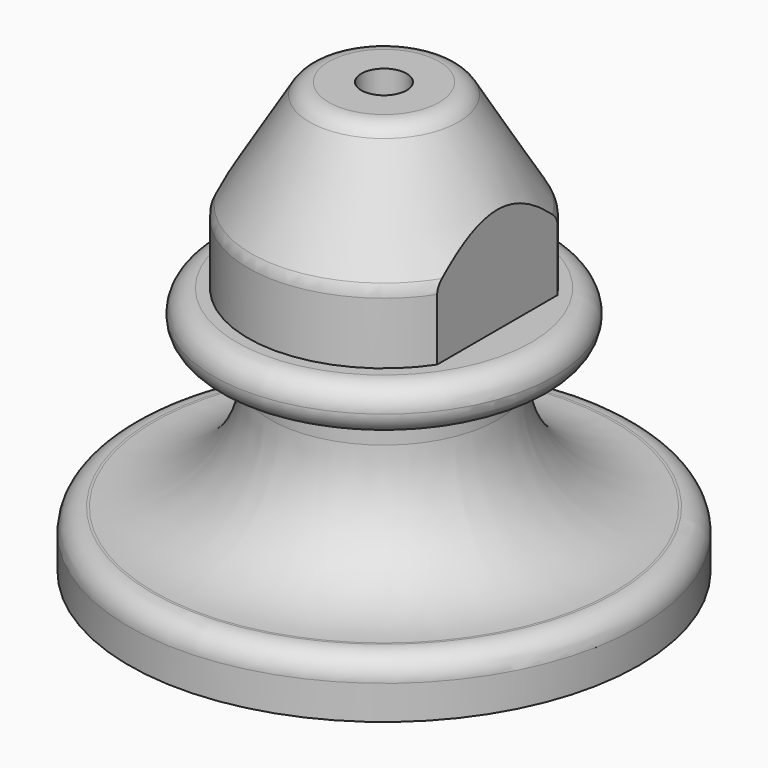
from build123d import *

# Parameters (mm, degrees)
F2_R     = 2
F3_R     = 2
F5_DEPTH = 16
F6_R     = 1.99999


# Not quite as in the source:
# - a fillet or chamfer is up to 0.001 mm smaller than in the source, because OpenCascade refuses the exact size


with BuildPart() as f1:
    # F0 (on Front) → F1 (revolve)
    with BuildSketch(Plane.XZ):
        with BuildLine():
            Line((19.5, 2.4493911769), (19.5, 0))
            Line((19.5, 0), (22.5, 0))
            Line((22.5, 0), (22.5, 5))
            Line((22.5, 5), (20.3029489522, 5))
            ThreePointArc((20.3029489522, 5), (13.036864554, 7.8180327534), (10, 14.9954100432))
            Line((10, 14.9954100432), (10, 18))
            Line((10, 18), (15, 18))
            Line((15, 18), (15, 22))
            Line((15, 22), (12, 22))
            Line((12, 22), (12, 28))
            Line((12, 28), (6, 38))
            Line((6, 38), (2, 38))
            Line((2, 38), (2, 25))
            Line((2, 25), (7, 25))
            Line((7, 25), (7, 14.6953836083))
            ThreePointArc((7, 14.6953836083), (10.6768777456, 5.9458931856), (19.5, 2.4493911769))
        make_face()
    revolve(axis=Axis((0, 0, 19), (0, 0, 1)))

    # F2
    f2_edges = [f1.edges().sort_by_distance(p)[0] for p in [
        (-6, 0, 38),
        (-12, 0, 28),
        (-15, 0, 22),
        (-22.5, 0, 5),
    ]]
    fillet(f2_edges, radius=F2_R)

    # F3
    f3_edges = [f1.edges().sort_by_distance(p)[0] for p in [
        (-7, 0, 25),
        (-19.5, 0, 2.449391),
    ]]
    fillet(f3_edges, radius=F3_R)

    # F4 (on face) → F5 (cut)
    with BuildSketch(Plane.XY.offset(38)):
        with BuildLine():
            Line((-10, -11.7565038997), (-10, 11.7565038997))
            ThreePointArc((-10, 11.7565038997), (-15.4342276756, 0), (-10, -11.7565038997))
        make_face()
        with BuildLine():
            ThreePointArc((10, -11.7565038997), (14.0099546876, -6.4758438518), (15.4342276756, 0))
            ThreePointArc((15.4342276756, 0), (14.0099546876, 6.4758438518), (10, 11.7565038997))
            Line((10, 11.7565038997), (10, -11.7565038997))
        make_face()
    extrude(amount=-F5_DEPTH, mode=Mode.SUBTRACT)

    # F6 (radius 2 in the source; OpenCascade refuses exactly that, so slightly less here)
    f6_edges = [f1.edges().sort_by_distance(p)[0] for p in [
        (-15, 0, 18),
    ]]
    fillet(f6_edges, radius=F6_R)


solid = f1.part
